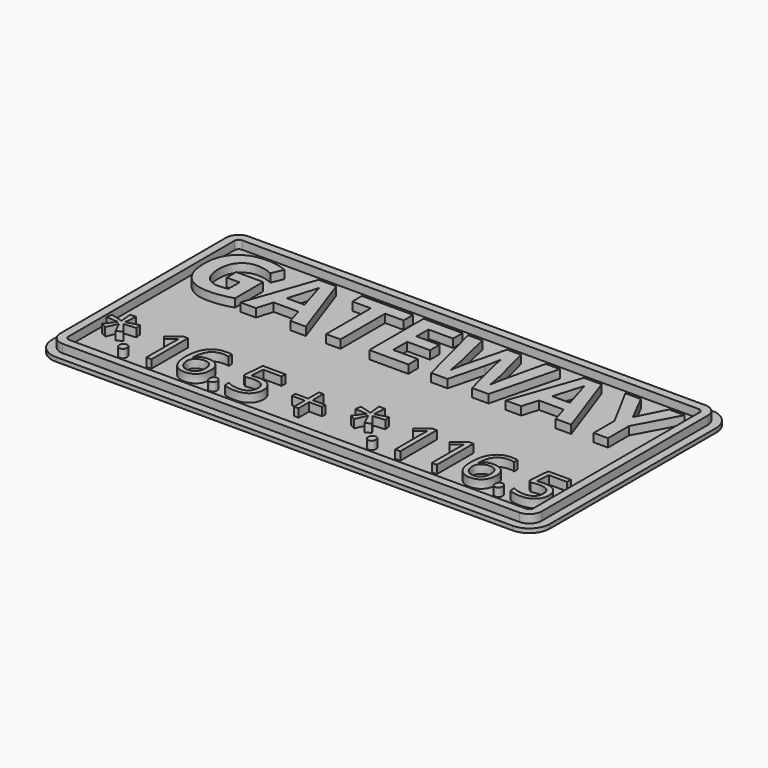
from build123d import *

# Parameters (mm, degrees)
F3_DEPTH       = 1
F4_TEXT_SIZE   = 22.8622460371
F4_TEXT_SIZE_2 = 15.4087577119
F5_DEPTH       = 2


# Not quite as in the source:
# - Text() gives the source's letters only with a copy of the font that has no kerning and outlines rounded to 1/6400 em; it was checked with that copy


with BuildPart() as f3:
    # F2 (on Top) → F3 (new body)
    with BuildSketch(Plane.XY):
        with BuildLine():
            Line((55, 30), (-55, 30))
            ThreePointArc((-55, 30), (-58.5355339059, 28.5355339059), (-60, 25))
            Line((-60, 25), (-60, -25))
            ThreePointArc((-60, -25), (-58.5355339059, -28.5355339059), (-55, -30))
            Line((-55, -30), (55, -30))
            ThreePointArc((55, -30), (58.5355339059, -28.5355339059), (60, -25))
            Line((60, -25), (60, 25))
            ThreePointArc((60, 25), (58.5355339059, 28.5355339059), (55, 30))
        make_face()
    extrude(amount=F3_DEPTH)

    # F4 (on face) → F5 (join)
    with BuildSketch(Plane.XY.offset(1)):
        with BuildLine():
            Line((55, 28), (-55, 28))
            ThreePointArc((-55, 28), (-57.1213203436, 27.1213203436), (-58, 25))
            Line((-58, 25), (-58, -25))
            ThreePointArc((-58, -25), (-57.1213203436, -27.1213203436), (-55, -28))
            Line((-55, -28), (55, -28))
            ThreePointArc((55, -28), (57.1213203436, -27.1213203436), (58, -25))
            Line((58, -25), (58, 25))
            ThreePointArc((58, 25), (57.1213203436, 27.1213203436), (55, 28))
        make_face()
        with BuildLine():
            ThreePointArc((-56, 25), (-55.7071067812, 25.7071067812), (-55, 26))
            Line((-55, 26), (55, 26))
            ThreePointArc((55, 26), (55.7071067812, 25.7071067812), (56, 25))
            Line((56, 25), (56, -25))
            ThreePointArc((56, -25), (55.7071067812, -25.7071067812), (55, -26))
            Line((55, -26), (-55, -26))
            ThreePointArc((-55, -26), (-55.7071067812, -25.7071067812), (-56, -25))
            Line((-56, -25), (-56, 25))
        make_face(mode=Mode.SUBTRACT)
        with Locations((-56, 6.050313618)):
            Text('GATEWAY', F4_TEXT_SIZE, font='Open Sans', font_style=FontStyle.BOLD, text_align=(TextAlign.LEFT, TextAlign.BOTTOM))
        with Locations((-56, -22.5111307647)):
            Text('*.16.5 + *.116.5', F4_TEXT_SIZE_2, font='Open Sans', text_align=(TextAlign.LEFT, TextAlign.BOTTOM))
    extrude(amount=F5_DEPTH)


solid = f3.part
